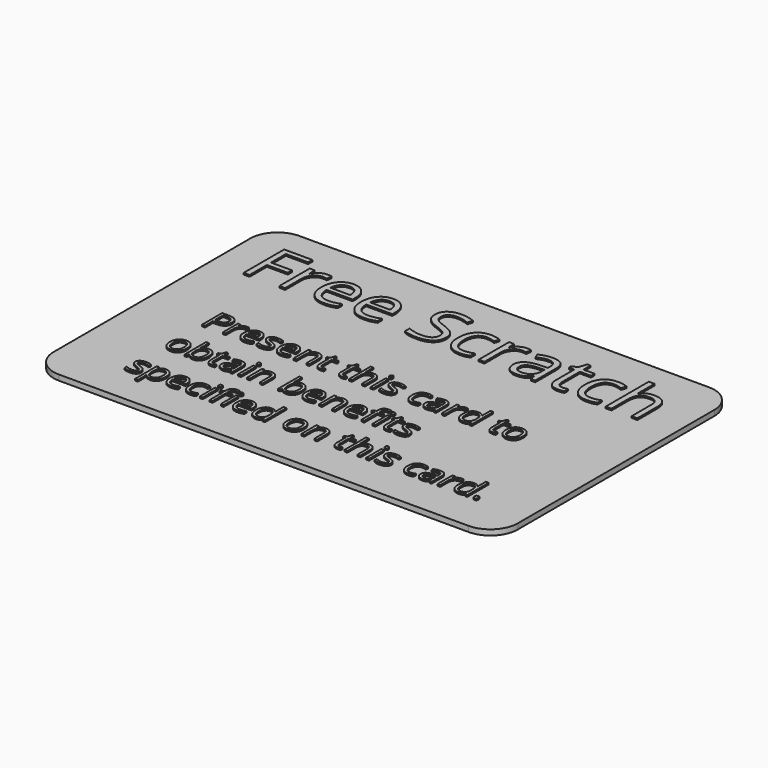
from build123d import *

# Parameters (mm, degrees)
F0_W           = 85
F0_H           = 55
F1_DEPTH       = 1
F2_R           = 5
F3_TEXT_SIZE   = 12.9699747688
F3_TEXT_SIZE_2 = 6.4479672195
F4_DEPTH       = 0.3


# Not quite as in the source:
# - Text() gives the source's letters only with a copy of the font that has no kerning and outlines rounded to 1/6400 em; it was checked with that copy


with BuildPart() as f1:
    # F0 (on Top) → F1 (new body)
    with BuildSketch(Plane.XY):
        with Locations((1.3076374307, -1.5492540755)):
            Rectangle(F0_W, F0_H)
    extrude(amount=F1_DEPTH)

    # F2
    f2_edges = [f1.edges().sort_by_distance(p)[0] for p in [
        (43.807637, -29.049254, 0.5),
        (43.807637, 25.950746, 0.5),
        (-41.192363, 25.950746, 0.5),
        (-41.192363, -29.049254, 0.5),
    ]]
    fillet(f2_edges, radius=F2_R)

    # F3 (on face) → F4 (join)
    with BuildSketch(Plane.XY.offset(1)):
        with Locations((-36.1923625693, 11.612364091)):
            Text('Free Scratch', F3_TEXT_SIZE, font='Open Sans', text_align=(TextAlign.LEFT, TextAlign.BOTTOM))
        with Locations((-30.1710683852, -4.642536398)):
            Text('Present this card to', F3_TEXT_SIZE_2, font='Open Sans', text_align=(TextAlign.LEFT, TextAlign.BOTTOM))
        with Locations((-30.1710683852, -13.4117718165)):
            Text('obtain benefits', F3_TEXT_SIZE_2, font='Open Sans', text_align=(TextAlign.LEFT, TextAlign.BOTTOM))
        with Locations((-30.1710683852, -22.181007235)):
            Text('specified on this card.', F3_TEXT_SIZE_2, font='Open Sans', text_align=(TextAlign.LEFT, TextAlign.BOTTOM))
    extrude(amount=F4_DEPTH)


solid = f1.part
